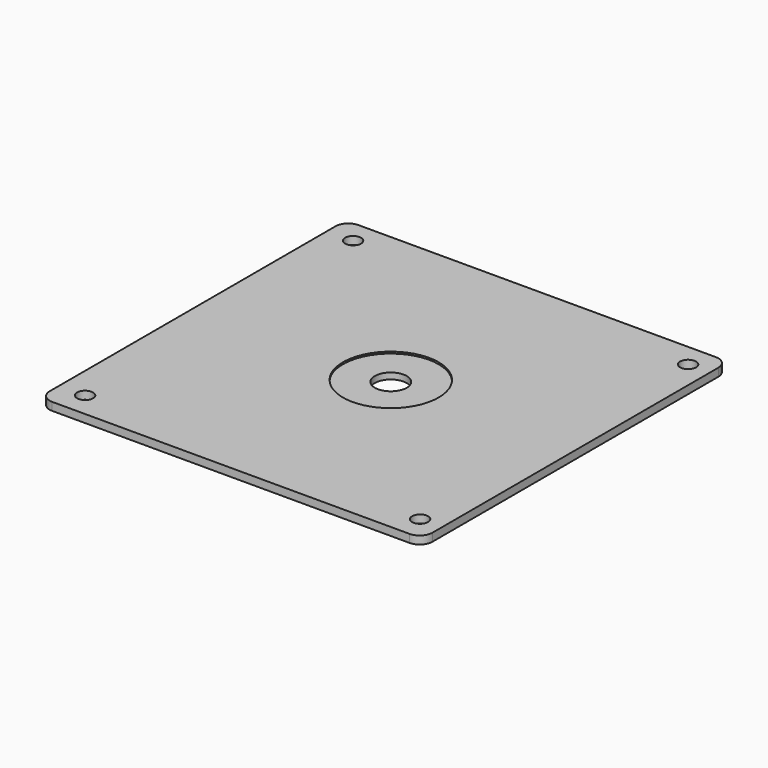
from build123d import *

# Parameters (mm, degrees)
F0_W     = 152.4
F0_H     = 152.4
F0_R     = 3.175
F0_R_2   = 6.35
F1_DEPTH = 3.175
F2_R     = 5.08
F3_R     = 19.044803008
F3_R_2   = 6.35
F4_DEPTH = 0.7055555556


# Not quite as in the source:
# - a length typed as a fraction of an inch, garbled in the dataset ("3 / 203.2 mm" for 3/8 in), is restored


with BuildPart() as f1:
    # F0 (on Top) → F1 (new body)
    with BuildSketch(Plane.XY):
        with Locations((-1.8146978691, -1.1040684107)):
            Rectangle(F0_W, F0_H)
        with Locations((-67.6762834191, -67.5093614922)):
            Circle(F0_R, mode=Mode.SUBTRACT)
        with Locations((65.6737165809, -67.5093614922)):
            Circle(F0_R, mode=Mode.SUBTRACT)
        with Locations((-67.6762834191, 65.8406385078)):
            Circle(F0_R, mode=Mode.SUBTRACT)
        Circle(F0_R_2, mode=Mode.SUBTRACT)
        with Locations((65.6737165809, 65.8406385078)):
            Circle(F0_R, mode=Mode.SUBTRACT)
    extrude(amount=F1_DEPTH)

    # F2
    f2_edges = [f1.edges().sort_by_distance(p)[0] for p in [
        (74.385302, 75.095932, 1.5875),
        (-78.014698, 75.095932, 1.5875),
        (74.385302, -77.304068, 1.5875),
        (-78.014698, -77.304068, 1.5875),
    ]]
    fillet(f2_edges, radius=F2_R)

    # F3 (on face) → F4 (cut)
    with BuildSketch(Plane.XY.offset(3.175)):
        Circle(F3_R)
        Circle(F3_R_2, mode=Mode.SUBTRACT)
    extrude(amount=-F4_DEPTH, mode=Mode.SUBTRACT)


solid = f1.part
